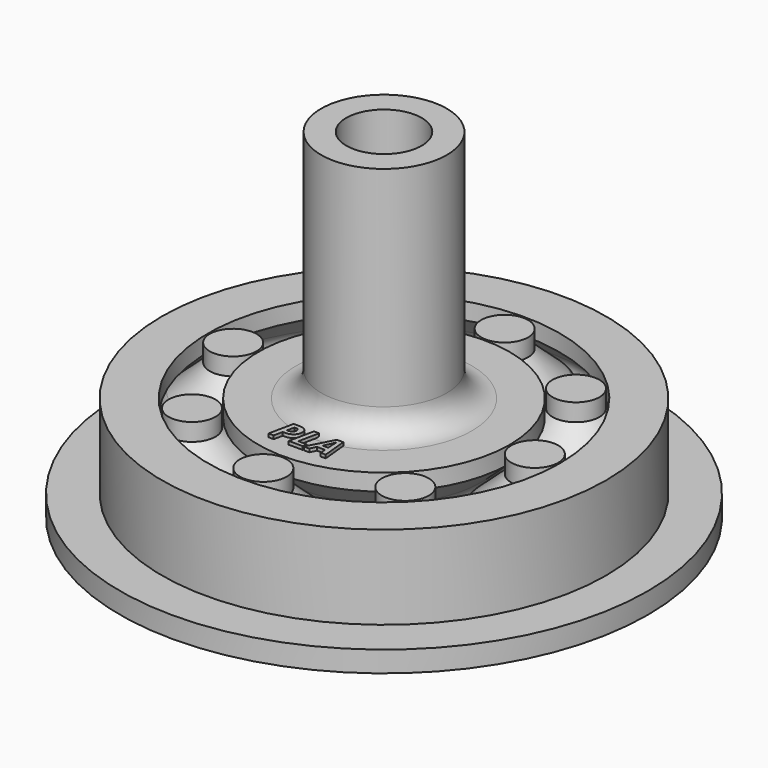
from build123d import *

# Parameters (mm, degrees)
F0_R          = 26.5
F1_DEPTH      = 38
F2_R          = 31.5000008196
F3_DEPTH      = 2.5
F5_D          = 9
F7_R          = 26.5
F7_R_2        = 7.5
F8_DEPTH      = 28.001
F14_COUNT     = 8
F15_R         = 3
F16_TEXT_SIZE = 4.1666666667
F17_DEPTH     = 0.4


# Not quite as in the source:
# - Text() gives the source's letters only with a copy of the font that has no kerning and outlines rounded to 1/6400 em; it was checked with that copy


with BuildPart() as f1:
    # F0 (on Top) → F1 (new body)
    with BuildSketch(Plane.XY):
        Circle(F0_R)
    extrude(amount=F1_DEPTH)

    # F2 (on Top) → F3 (join)
    with BuildSketch(Plane.XY):
        Circle(F2_R)
    extrude(amount=-F3_DEPTH)

    # F5 (through all)
    with Locations(Plane(origin=(0, 0, -2.5), x_dir=(1, 0, 0), z_dir=(0, 0, -1))):
        with Locations((0, 0)):
            Hole(F5_D / 2)

    # F7 (on offset) → F8 (cut, through all)
    with BuildSketch(Plane.XY.offset(10)):
        Circle(F7_R)
        Circle(F7_R_2, mode=Mode.SUBTRACT)
    extrude(amount=F8_DEPTH, mode=Mode.SUBTRACT)

    # F10 (on Front) → F11 (revolve, cut)
    with BuildSketch(Plane.XZ):
        with BuildLine():
            Line((15, 8), (11.6597938144, 4.9845360825))
            ThreePointArc((11.6597938144, 4.9845360825), (11.0020629196, 3.4091846782), (11.8, 1.9))
            Line((11.8, 1.9), (15, -0.5))
            Line((15, -0.5), (15, -2.5))
            Line((15, -2.5), (21, -2.5))
            Line((21, -2.5), (21, -0.5))
            Line((21, -0.5), (24.2, 1.9))
            ThreePointArc((24.2, 1.9), (24.9979370804, 3.4091846782), (24.3402061856, 4.9845360825))
            Line((24.3402061856, 4.9845360825), (21, 8))
            Line((21, 8), (21, 10))
            Line((21, 10), (15, 10))
            Line((15, 10), (15, 8))
        make_face()
    revolve(axis=Axis((0, 0, 30.2871484309), (0, 0, 1)), mode=Mode.SUBTRACT)

    # F15
    f15_edges = [f1.edges().sort_by_distance(p)[0] for p in [
        (-7.5, 0, 10),
    ]]
    fillet(f15_edges, radius=F15_R)

    # F16 (on face) → F17 (join)
    with BuildSketch(Plane.XY.offset(10)):
        with Locations((-3.6061197917, -12.8613335837)):
            Text('PLA', F16_TEXT_SIZE, font='Open Sans', font_style=FontStyle.BOLDITALIC, text_align=(TextAlign.LEFT, TextAlign.BOTTOM))
    extrude(amount=F17_DEPTH)


with BuildPart() as f13:
    # F12 (on Front) → F13 (revolve)
    with BuildSketch(Plane.XZ):
        with BuildLine():
            Line((15.2, 7.9111111111), (11.793814433, 4.8360824742))
            ThreePointArc((11.793814433, 4.8360824742), (11.2334194728, 3.1547562586), (12.3855718597, 1.8081140522))
            Line((12.3855718597, 1.8081140522), (15.2, -0.4111111111))
            Line((15.2, -0.4111111111), (15.2, -2.5))
            Line((15.2, -2.5), (18, -2.5))
            Line((18, -2.5), (18, 10))
            Line((18, 10), (15.2, 10))
            Line((15.2, 10), (15.2, 7.9111111111))
        make_face()
    revolve(axis=Axis((18, 0, 3.4731910564), (0, 0, -1)))


with BuildPart() as f14_1:
    # F14: instance of F13
    add(f13.part.rotate(Axis((0, 0, 30.2871484309), (0, 0, 1)), 1 * 360 / F14_COUNT))


with BuildPart() as f14_2:
    # F14: instance of F13
    add(f13.part.rotate(Axis((0, 0, 30.2871484309), (0, 0, 1)), 2 * 360 / F14_COUNT))


with BuildPart() as f14_3:
    # F14: instance of F13
    add(f13.part.rotate(Axis((0, 0, 30.2871484309), (0, 0, 1)), 3 * 360 / F14_COUNT))


with BuildPart() as f14_4:
    # F14: instance of F13
    add(f13.part.rotate(Axis((0, 0, 30.2871484309), (0, 0, 1)), 4 * 360 / F14_COUNT))


with BuildPart() as f14_5:
    # F14: instance of F13
    add(f13.part.rotate(Axis((0, 0, 30.2871484309), (0, 0, 1)), 5 * 360 / F14_COUNT))


with BuildPart() as f14_6:
    # F14: instance of F13
    add(f13.part.rotate(Axis((0, 0, 30.2871484309), (0, 0, 1)), 6 * 360 / F14_COUNT))


with BuildPart() as f14_7:
    # F14: instance of F13
    add(f13.part.rotate(Axis((0, 0, 30.2871484309), (0, 0, 1)), 7 * 360 / F14_COUNT))


solid = Compound([f1.part, f13.part, f14_1.part, f14_2.part, f14_3.part, f14_4.part, f14_5.part, f14_6.part, f14_7.part])
